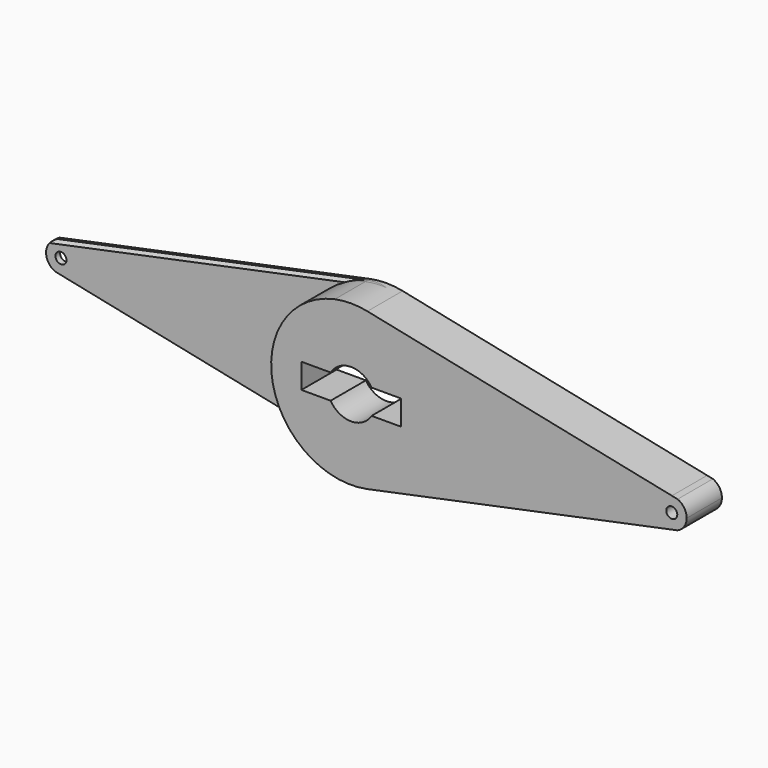
from build123d import *

# Parameters (mm, degrees)
F0_R        = 9.525
F1_DEPTH    = 76.2
F2_DEPTH    = 10.16
F3_T4_DEPTH = 600.435352042
F3_S5_R     = 138.2955463349
F3_T6_DEPTH = 303


# Not quite as in the source:
# - a fillet or chamfer that OpenCascade refuses, or shapes differently, is made with other operations: its cross-section is extruded or revolved along the edge and cut away or added


with BuildPart() as f1:
    # F0 (on Front) → F1 (new body)
    with BuildSketch(Plane.XZ):
        with BuildLine():
            ThreePointArc((28.1677821814, -135.396581135), (107.2873174282, -87.2644810626), (138.2955463349, 0))
            ThreePointArc((138.2955463349, 0), (107.2890589283, 87.2623399316), (28.1731863292, 135.3954567484))
            ThreePointArc((28.1731863292, 135.3954567484), (0, 138.2955463349), (-28.1731863292, 135.3954567484))
            ThreePointArc((-28.1731863292, 135.3954567484), (-138.2955463073, -0.0027599392), (-28.1677821814, -135.396581135))
            ThreePointArc((-28.1677821814, -135.396581135), (0, -138.2955463349), (28.1677821814, -135.396581135))
        make_face()
        with BuildLine():
            ThreePointArc((-35.4519361343, 21.4876397772), (0, 41.4554995009), (35.4519361343, 21.4876397772))
            Line((35.4519361343, 21.4876397772), (85.9505591086, 21.4876397772))
            Line((85.9505591086, 21.4876397772), (85.9505591086, -21.4876397772))
            Line((85.9505591086, -21.4876397772), (35.4519361343, -21.4876397772))
            ThreePointArc((35.4519361343, -21.4876397772), (0, -41.4554995009), (-35.4519361343, -21.4876397772))
            Line((-35.4519361343, -21.4876397772), (-85.9505591086, -21.4876397772))
            Line((-85.9505591086, -21.4876397772), (-85.9505591086, 21.4876397772))
            Line((-85.9505591086, 21.4876397772), (-35.4519361343, 21.4876397772))
        make_face(mode=Mode.SUBTRACT)
        with BuildLine():
            ThreePointArc((28.1731863292, 135.3954567484), (107.2890589283, 87.2623399316), (138.2955463349, 0))
            ThreePointArc((138.2955463349, 0), (107.2873174282, -87.2644810626), (28.1677821814, -135.396581135))
            Line((28.1677821814, -135.396581135), (555.0553956372, -25.7833589585))
            ThreePointArc((555.0553956372, -25.7833589585), (528.9648763124, -0.0553010475), (554.9447987454, 25.7844317855))
            Line((554.9447987454, 25.7844317855), (28.1731863292, 135.3954567484))
        make_face()
        with BuildLine():
            Line((564.856504828, 23.7219966861), (554.9447987454, 25.7844317855))
            ThreePointArc((554.9447987454, 25.7844317855), (528.9648763124, -0.0553010475), (555.0553956372, -25.7833589585))
            Line((555.0553956372, -25.7833589585), (564.7527625578, -23.7659275222))
            ThreePointArc((564.7527625578, -23.7659275222), (576.2301870088, -14.2644938792), (580.5351524758, 0))
            ThreePointArc((580.5351524758, 0), (576.2612979363, 14.2175342345), (564.856504828, 23.7219966861))
        make_face()
        with Locations((554.7499847432, 0)):
            Circle(F0_R, mode=Mode.SUBTRACT)
    extrude(amount=F1_DEPTH)

    # F0 (on Front) → F2 (join)
    with BuildSketch(Plane.XZ):
        with BuildLine():
            ThreePointArc((-28.1677821814, -135.396581135), (-138.2955463073, -0.0027599392), (-28.1731863292, 135.3954567484))
            Line((-28.1731863292, 135.3954567484), (-554.9447987454, 25.7844317855))
            ThreePointArc((-554.9447987454, 25.7844317855), (-536.5861255267, 18.3016145015), (-528.9648170106, 0))
            ThreePointArc((-528.9648170106, 0), (-536.6254184882, -18.3405281566), (-555.0553956372, -25.7833589585))
            Line((-555.0553956372, -25.7833589585), (-28.1677821814, -135.396581135))
        make_face()
        with BuildLine():
            ThreePointArc((-528.9648170106, 0), (-536.5861255267, 18.3016145015), (-554.9447987454, 25.7844317855))
            Line((-554.9447987454, 25.7844317855), (-564.856504828, 23.7219966861))
            ThreePointArc((-564.856504828, 23.7219966861), (-580.5350909463, -0.056330225), (-564.7527625578, -23.7659275222))
            Line((-564.7527625578, -23.7659275222), (-555.0553956372, -25.7833589585))
            ThreePointArc((-555.0553956372, -25.7833589585), (-536.6254184882, -18.3405281566), (-528.9648170106, 0))
        make_face()
        with Locations((-554.7499847432, 0)):
            Circle(F0_R, mode=Mode.SUBTRACT)
    extrude(amount=F2_DEPTH)

    # F3: chamfer of 5.08 on 1 edges, made by hand


with BuildPart() as f3_tool2:
    # F3_s3 → F3_t4 (new body)
    with BuildSketch(Plane(origin=(38.3705740236, 0, 7.9841772943), x_dir=(0, 1, 0), z_dir=(-0.9790297688, 0, -0.2037172351))):
        Polygon((-5.08, -138.2955463349), (-10.16, -133.2155463349), (-10.16, -138.2955463349), align=None)
    extrude(amount=F3_T4_DEPTH)

    # F3_s5 → F3_t6 (cut, symmetric)
    with BuildSketch(Plane.XZ.offset(7.6)):
        Circle(F3_S5_R)
    extrude(amount=F3_T6_DEPTH, both=True, mode=Mode.SUBTRACT)


with BuildPart() as f1_1:
    add(f1.part)

    # F3_t1: cut F3_tool2
    add(f3_tool2.part, mode=Mode.SUBTRACT)


solid = f1_1.part
